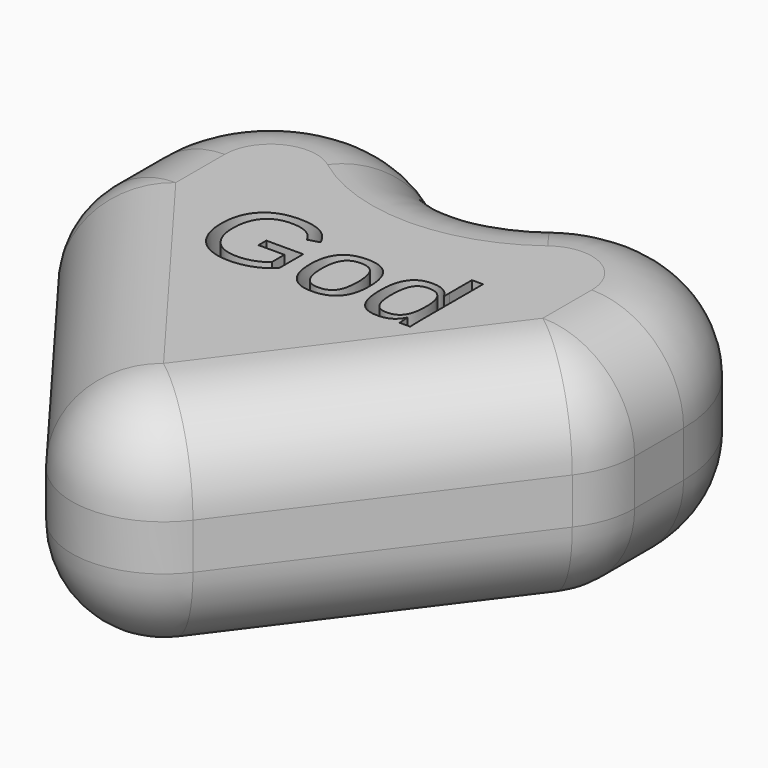
from build123d import *

# Parameters (mm, degrees)
F1_DEPTH     = 12.5
F2_R         = 10
F4_TEXT_SIZE = 13.7605393926
F5_DEPTH     = 5
F3_R         = 3.8513157681
F3_R_2       = 2.6013157681
F6_DEPTH     = 1


# Not quite as in the source:
# - Text() gives the source's letters only with a copy of the font that has no kerning and outlines rounded to 1/6400 em; it was checked with that copy


with BuildPart() as f1:
    # F0 (on Top) → F1 (new body, symmetric)
    with BuildSketch(Plane.XY):
        with BuildLine():
            Line((-30, 10), (-30, 0))
            Line((-30, 0), (0, -40))
            Line((0, -40), (30, 0))
            Line((30, 0), (30, 10))
            ThreePointArc((30, 10), (15, 25), (0, 10))
            ThreePointArc((0, 10), (-15, 25), (-30, 10))
        make_face()
    extrude(amount=F1_DEPTH, both=True)

    # F2
    f2_edges = [f1.edges().sort_by_distance(p)[0] for p in [
        (30, 5, -12.5),
        (-30, 5, -12.5),
        (-15, -20, -12.5),
        (15, -20, -12.5),
        (15, 25, -12.5),
        (-15, 25, -12.5),
        (-30, 5, 12.5),
        (-15, -20, 12.5),
        (15, -20, 12.5),
        (30, 5, 12.5),
        (15, 25, 12.5),
        (-15, 25, 12.5),
        (30, 10, 0),
        (30, 0, 0),
        (0, -40, 0),
        (-30, 10, 0),
        (-30, 0, 0),
        (0, 10, 0),
    ]]
    fillet(f2_edges, radius=F2_R)

    # F4 (on face) → F5 (cut)
    with BuildSketch(Plane.XY.offset(12.5)):
        with Locations((-12.9674943164, -4.9367714673)):
            Text('God', F4_TEXT_SIZE, font='Arimo', text_align=(TextAlign.LEFT, TextAlign.BOTTOM))
    extrude(amount=-F5_DEPTH, mode=Mode.SUBTRACT)

    # F3 (on Top) → F6 (join, symmetric)
    with BuildSketch(Plane.XY):
        with Locations((0, 21.951623261)):
            Circle(F3_R)
        with Locations((0, 21.951623261)):
            Circle(F3_R_2, mode=Mode.SUBTRACT)
    extrude(amount=F6_DEPTH, both=True)


solid = f1.part
